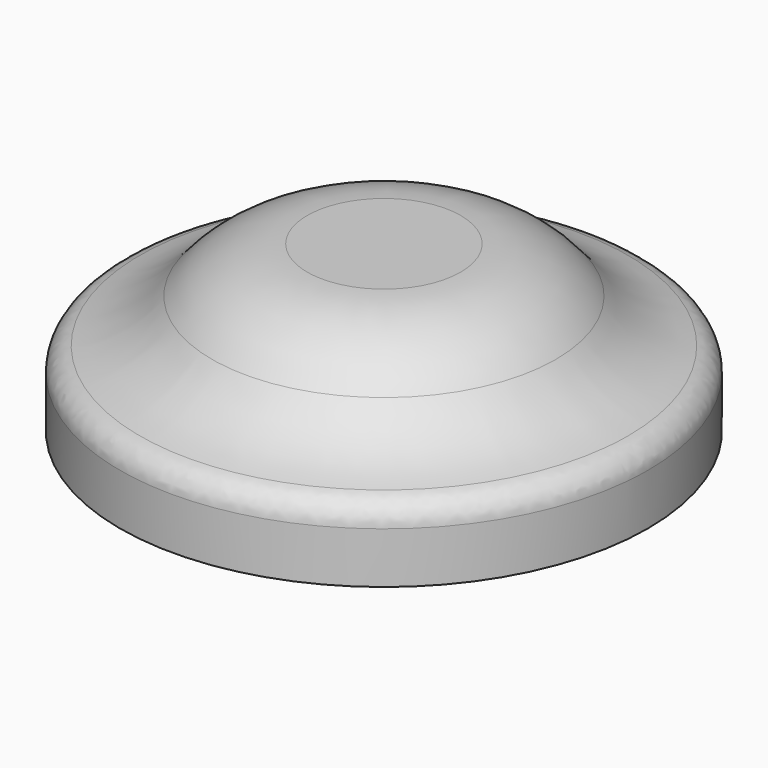
from build123d import *

# Parameters (mm, degrees)
F4_R     = 1
F5_R     = 5.9
F6_DEPTH = 2.85
F7_SIZE2 = 1
F7_SIZE  = 5


# Not quite as in the source:
# - a fillet or chamfer that OpenCascade refuses, or shapes differently, is made with other operations: its cross-section is extruded or revolved along the edge and cut away or added


with BuildPart() as f1:
    # F0 (on Front) → F1 (revolve)
    with BuildSketch(Plane.XZ):
        Polygon((8, 13.6877541882), (0, 13.6877541882), (0, 6.9177541882), (10.85, 6.9177541882), (10.85, 9.9177541882), (8, 9.9177541882), align=None)
    revolve(axis=Axis((0, 0, 10.3027541882), (0, 0, 1)))

    # F2: fillet of radius 5 on 1 edges, made by hand

    # F2_s1 → F2_t2 (revolve, cut)
    with BuildSketch(Plane.XZ):
        with BuildLine():
            ThreePointArc((3.1536508586, 13.6877541882), (6.2236671452, 12.6342716403), (8, 9.9177541882))
            Line((8, 9.9177541882), (8, 13.6877541882))
            Line((8, 13.6877541882), (3.1536508586, 13.6877541882))
        make_face()
    revolve(axis=Axis((0, 0, 13.6877541882), (0, 0, 1)), mode=Mode.SUBTRACT)

    # F3: fillet of radius 5 on 1 edges, made by hand

    # F3_s1 → F3_t2 (revolve)
    with BuildSketch(Plane.XZ):
        with BuildLine():
            ThreePointArc((7.0654038886, 11.8019456133), (8.7487622666, 10.4401726424), (10.85, 9.9177541882))
            Line((10.85, 9.9177541882), (8, 9.9177541882))
            ThreePointArc((8, 9.9177541882), (7.6328955207, 10.9095478909), (7.0654038886, 11.8019456133))
        make_face()
    revolve(axis=Axis((0, 0, 9.9177541882), (0, 0, 1)))

    # F4
    f4_edges = [f1.edges().sort_by_distance(p)[0] for p in [
        (-10.85, 0, 9.917754),
    ]]
    fillet(f4_edges, radius=F4_R)

    # F5 (on face) → F6 (cut)
    with BuildSketch(Plane(origin=(0, 0, 6.9177541882), x_dir=(1, 0, 0), z_dir=(0, 0, -1))):
        Circle(F5_R)
    extrude(amount=-F6_DEPTH, mode=Mode.SUBTRACT)

    # F7
    f7_edges = [f1.edges().sort_by_distance(p)[0] for p in [
        (-5.9, 0, 9.767754),
    ]]
    f7_side = f1.faces().sort_by_distance((0, 0, 9.767754))[0]
    chamfer(f7_edges, length=F7_SIZE, length2=F7_SIZE2, reference=f7_side)


solid = f1.part
